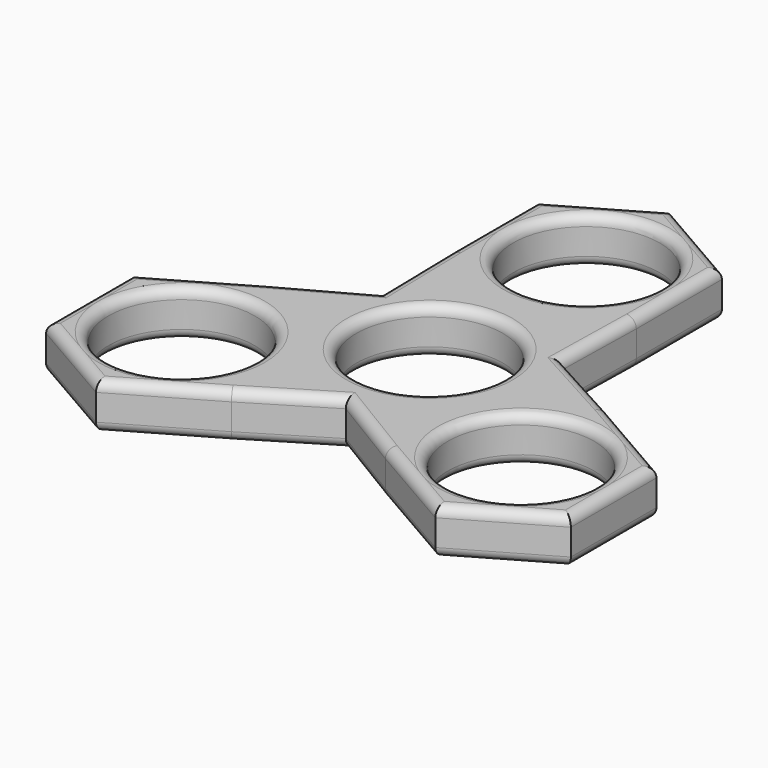
from build123d import *

# Parameters (mm, degrees)
F0_R         = 11.2
F1_DEPTH     = 7
F2_T1_DEPTH  = 23.8532758355
F2_T3_DEPTH  = 23.8532758355
F2_T5_DEPTH  = 23.8532758355
F2_T7_DEPTH  = 23.8532758355
F2_T9_DEPTH  = 23.8532758355
F2_T11_DEPTH = 23.8532758355
F2_T13_DEPTH = 23.8532758355
F2_T15_DEPTH = 23.8532758355
F2_T17_DEPTH = 23.8532758355
F2_T19_DEPTH = 23.8532758355
F2_T24_DEPTH = 21.2490117481
F2_T29_DEPTH = 21.2494848071
F2_T34_DEPTH = 21.2494848071
F2_T39_DEPTH = 21.2490117481
F2_T44_DEPTH = 21.249
F2_T49_DEPTH = 21.249
F2_T63_DEPTH = 21.2490117481
F2_T67_DEPTH = 21.2494848071
F2_T74_DEPTH = 21.2494848071
F2_T78_DEPTH = 21.2490117481
F2_T85_DEPTH = 21.249
F2_T89_DEPTH = 21.249
F3_T1_DEPTH  = 23.8532758355
F3_T3_DEPTH  = 23.8532758355
F3_T5_DEPTH  = 23.8532758355
F3_T7_DEPTH  = 23.8532758355
F3_T9_DEPTH  = 23.8532758355
F3_T11_DEPTH = 23.8532758355
F3_T13_DEPTH = 23.8532758355
F3_T15_DEPTH = 23.8532758355
F3_T17_DEPTH = 23.8532758355
F3_T19_DEPTH = 23.8532758355
F3_T24_DEPTH = 21.2490117481
F3_T29_DEPTH = 21.2494848071
F3_T34_DEPTH = 21.2494848071
F3_T39_DEPTH = 21.2490117481
F3_T44_DEPTH = 21.249
F3_T49_DEPTH = 21.249
F3_T63_DEPTH = 21.2494848071
F3_T67_DEPTH = 21.2490117481
F3_T74_DEPTH = 21.2490117481
F3_T78_DEPTH = 21.2494848071
F3_T85_DEPTH = 21.249
F3_T89_DEPTH = 21.249


# Not quite as in the source:
# - a fillet or chamfer that OpenCascade refuses, or shapes differently, is made with other operations: its cross-section is extruded or revolved along the edge and cut away or added


with BuildPart() as f1:
    # F0 (on Top) → F1 (new body)
    with BuildSketch(Plane.XY):
        Polygon((14.1623523086, 21.7544313529), (14.1623523086, 38.1077071884), (0, 46.2843451062), (-14.1623523086, 38.1077071884), (-14.1623523086, 21.7544313529), (-13.8703454286, 8.0080476669), (-25.9207897747, 1.388220244), (-40.0831420834, -6.7884176737), (-40.0831420834, -23.1416935092), (-25.9207897747, -31.318331427), (-11.7584374661, -23.1416935092), (0, -16.0160953339), (11.7584374661, -23.1416935092), (25.9207897747, -31.318331427), (40.0831420834, -23.1416935092), (40.0831420834, -6.7884176737), (25.9207897747, 1.388220244), (13.8703454286, 8.0080476669), align=None)
        with Locations((-25.9207897747, -14.9650555915)):
            Circle(F0_R, mode=Mode.SUBTRACT)
        Circle(F0_R, mode=Mode.SUBTRACT)
        with Locations((25.9207897747, -14.9650555915)):
            Circle(F0_R, mode=Mode.SUBTRACT)
        with Locations((0, 29.9310692707)):
            Circle(F0_R, mode=Mode.SUBTRACT)
    extrude(amount=F1_DEPTH)

    # F2: fillet of radius 1.5 on 22 edges, made by hand

    # F2_s2 → F2_t1 (cut)
    with BuildSketch(Plane(origin=(36.2494229052, -20.9286140723, 0), x_dir=(0, 0, 1), z_dir=(-0.8660254038, 0.5, 0))):
        with BuildLine():
            ThreePointArc((5.5, 14.1626288847), (6.5606601718, 13.7232890565), (7, 12.6626288847))
            Line((7, 12.6626288847), (7, 14.1626288847))
            Line((7, 14.1626288847), (5.5, 14.1626288847))
        make_face()
    extrude(amount=F2_T1_DEPTH, mode=Mode.SUBTRACT)

    # F2_s4 → F2_t3 (cut)
    with BuildSketch(Plane.XZ.offset(-41.8577071884)):
        with BuildLine():
            ThreePointArc((14.1623523086, 5.5), (13.7230124804, 6.5606601718), (12.6623523086, 7))
            Line((12.6623523086, 7), (14.1623523086, 7))
            Line((14.1623523086, 7), (14.1623523086, 5.5))
        make_face()
        with BuildLine():
            ThreePointArc((-14.1623523086, 5.5), (-13.7230124804, 6.5606601718), (-12.6623523086, 7))
            Line((-12.6623523086, 7), (-14.1623523086, 7))
            Line((-14.1623523086, 7), (-14.1623523086, 5.5))
        make_face()
    extrude(amount=F2_T3_DEPTH, mode=Mode.SUBTRACT)

    # F2_s6 → F2_t5 (cut)
    with BuildSketch(Plane(origin=(-2.6317617569, 1.5194483588, 0), x_dir=(0, 0, 1), z_dir=(-0.8660254038, 0.5, 0))):
        with BuildLine():
            ThreePointArc((5.5, 40.0834186595), (6.5606601718, 39.6440788312), (7, 38.5834186595))
            Line((7, 38.5834186595), (7, 40.0834186595))
            Line((7, 40.0834186595), (5.5, 40.0834186595))
        make_face()
    extrude(amount=F2_T5_DEPTH, mode=Mode.SUBTRACT)

    # F2_s8 → F2_t7 (cut)
    with BuildSketch(Plane(origin=(23.2893045939, 13.4460862765, 0), x_dir=(0, 0, 1), z_dir=(-0.8660254038, -0.5, 0))):
        with BuildLine():
            ThreePointArc((5.5, 40.0834186595), (6.5606601718, 39.6440788312), (7, 38.5834186595))
            Line((7, 38.5834186595), (7, 40.0834186595))
            Line((7, 40.0834186595), (5.5, 40.0834186595))
        make_face()
    extrude(amount=F2_T7_DEPTH, mode=Mode.SUBTRACT)

    # F2_s10 → F2_t9 (cut)
    with BuildSketch(Plane(origin=(-15.5918800682, -9.0019761545, 0), x_dir=(0, 0, 1), z_dir=(-0.8660254038, -0.5, 0))):
        with BuildLine():
            ThreePointArc((5.5, 14.1626288847), (6.5606601718, 13.7232890565), (7, 12.6626288847))
            Line((7, 12.6626288847), (7, 14.1626288847))
            Line((7, 14.1626288847), (5.5, 14.1626288847))
        make_face()
    extrude(amount=F2_T9_DEPTH, mode=Mode.SUBTRACT)

    # F2_s12 → F2_t11 (cut)
    with BuildSketch(Plane.XZ.offset(3.0384176737)):
        with BuildLine():
            ThreePointArc((-40.0831420834, 5.5), (-39.6438022551, 6.5606601718), (-38.5831420834, 7))
            Line((-38.5831420834, 7), (-40.0831420834, 7))
            Line((-40.0831420834, 7), (-40.0831420834, 5.5))
        make_face()
        with BuildLine():
            ThreePointArc((40.0831420834, 5.5), (39.6438022551, 6.5606601718), (38.5831420834, 7))
            Line((38.5831420834, 7), (40.0831420834, 7))
            Line((40.0831420834, 7), (40.0831420834, 5.5))
        make_face()
    extrude(amount=F2_T11_DEPTH, mode=Mode.SUBTRACT)

    # F2_s14 → F2_t13 (cut)
    with BuildSketch(Plane(origin=(-23.2893045939, 13.4460862765, 0), x_dir=(0, 0, 1), z_dir=(0.8660254038, -0.5, 0))):
        with BuildLine():
            ThreePointArc((5.5, 40.0828655072), (6.5606601718, 39.643525679), (7, 38.5828655072))
            Line((7, 38.5828655072), (7, 40.0828655072))
            Line((7, 40.0828655072), (5.5, 40.0828655072))
        make_face()
    extrude(amount=F2_T13_DEPTH, mode=Mode.SUBTRACT)

    # F2_s16 → F2_t15 (cut)
    with BuildSketch(Plane(origin=(-36.2494229052, -20.9286140723, 0), x_dir=(0, 0, 1), z_dir=(0.8660254038, 0.5, 0))):
        with BuildLine():
            ThreePointArc((5.5, 14.1620757325), (6.5606601718, 13.7227359043), (7, 12.6620757325))
            Line((7, 12.6620757325), (7, 14.1620757325))
            Line((7, 14.1620757325), (5.5, 14.1620757325))
        make_face()
    extrude(amount=F2_T15_DEPTH, mode=Mode.SUBTRACT)

    # F2_s18 → F2_t17 (cut)
    with BuildSketch(Plane(origin=(15.5918800682, -9.0019761545, 0), x_dir=(0, 0, 1), z_dir=(0.8660254038, -0.5, 0))):
        with BuildLine():
            ThreePointArc((5.5, 14.1620757325), (6.5606601718, 13.7227359043), (7, 12.6620757325))
            Line((7, 12.6620757325), (7, 14.1620757325))
            Line((7, 14.1620757325), (5.5, 14.1620757325))
        make_face()
    extrude(amount=F2_T17_DEPTH, mode=Mode.SUBTRACT)

    # F2_s20 → F2_t19 (cut)
    with BuildSketch(Plane(origin=(2.6317617569, 1.5194483588, 0), x_dir=(0, 0, 1), z_dir=(0.8660254038, 0.5, 0))):
        with BuildLine():
            ThreePointArc((5.5, 40.0828655072), (6.5606601718, 39.643525679), (7, 38.5828655072))
            Line((7, 38.5828655072), (7, 40.0828655072))
            Line((7, 40.0828655072), (5.5, 40.0828655072))
        make_face()
    extrude(amount=F2_T19_DEPTH, mode=Mode.SUBTRACT)


with BuildPart() as f2_tool22:
    # F2_s23 → F2_t24 (new body)
    with BuildSketch(Plane(origin=(22.6127394317, -12.422150445, 0), x_dir=(0, 0, 1), z_dir=(-0.8764589461, 0.4814765995, 0))):
        with BuildLine():
            ThreePointArc((5.5, 13.696971769), (6.5606601718, 13.2576319408), (7, 12.196971769))
            Line((7, 12.196971769), (7, 13.696971769))
            Line((7, 13.696971769), (5.5, 13.696971769))
        make_face()
    extrude(amount=F2_T24_DEPTH)

    split(bisect_by=Plane(origin=(13.6940555403, -0.290895302, 0), x_dir=(0, 0, 1), z_dir=(0.9997744555, -0.0212376597, 0)), keep=Keep.TOP)


with BuildPart() as f1_1:
    add(f1.part)

    # F2_t21: cut F2_tool22
    add(f2_tool22.part, mode=Mode.SUBTRACT)


with BuildPart() as f2_tool27:
    # F2_s28 → F2_t29 (new body)
    with BuildSketch(Plane(origin=(0.0966486642, 4.5497887609, 0), x_dir=(0, 0, 1), z_dir=(0.0212376597, 0.9997744555, 0))):
        with BuildLine():
            ThreePointArc((5.5, 13.6971448564), (6.5606601718, 13.2578050282), (7, 12.1971448564))
            Line((7, 12.1971448564), (7, 13.6971448564))
            Line((7, 13.6971448564), (5.5, 13.6971448564))
        make_face()
    extrude(amount=F2_T29_DEPTH)

    split(bisect_by=Plane(origin=(6.5947713908, 12.0048334409, 0), x_dir=(0, 0, 1), z_dir=(0.4814765995, 0.8764589461, 0)), keep=Keep.TOP)


with BuildPart() as f1_2:
    add(f1_1.part)

    # F2_t26: cut F2_tool27
    add(f2_tool27.part, mode=Mode.SUBTRACT)


with BuildPart() as f2_tool32:
    # F2_s33 → F2_t34 (new body)
    with BuildSketch(Plane(origin=(-0.5479379924, 25.7944808629, 0), x_dir=(0, 0, 1), z_dir=(0.0212376597, -0.9997744555, 0))):
        with BuildLine():
            ThreePointArc((5.5, 13.6971448564), (6.5606601718, 13.2578050282), (7, 12.1971448564))
            Line((7, 12.1971448564), (7, 13.6971448564))
            Line((7, 13.6971448564), (5.5, 13.6971448564))
        make_face()
    extrude(amount=F2_T34_DEPTH)

    split(bisect_by=Plane(origin=(-6.5947713908, 12.0048334409, 0), x_dir=(0, 0, 1), z_dir=(-0.4814765995, 0.8764589461, 0)), keep=Keep.TOP)


with BuildPart() as f1_3:
    add(f1_2.part)

    # F2_t31: cut F2_tool32
    add(f2_tool32.part, mode=Mode.SUBTRACT)


with BuildPart() as f2_tool37:
    # F2_s38 → F2_t39 (new body)
    with BuildSketch(Plane(origin=(-3.9888529901, -2.1912485259, 0), x_dir=(0, 0, 1), z_dir=(-0.8764589461, -0.4814765995, 0))):
        with BuildLine():
            ThreePointArc((5.5, 13.696971769), (6.5606601718, 13.2576319408), (7, 12.196971769))
            Line((7, 12.196971769), (7, 13.696971769))
            Line((7, 13.696971769), (5.5, 13.696971769))
        make_face()
    extrude(amount=F2_T39_DEPTH)

    split(bisect_by=Plane(origin=(-13.6940555403, -0.290895302, 0), x_dir=(0, 0, 1), z_dir=(-0.9997744555, -0.0212376597, 0)), keep=Keep.TOP)


with BuildPart() as f1_4:
    add(f1_3.part)

    # F2_t36: cut F2_tool37
    add(f2_tool37.part, mode=Mode.SUBTRACT)


with BuildPart() as f2_tool42:
    # F2_s43 → F2_t44 (new body)
    with BuildSketch(Plane(origin=(-22.0643241976, -13.3709524497, 0), x_dir=(0, 0, 1), z_dir=(0.8552212864, 0.5182630137, 0))):
        with BuildLine():
            ThreePointArc((5.5, 13.6973056538), (6.5606601718, 13.2579658256), (7, 12.1973056538))
            Line((7, 12.1973056538), (7, 13.6973056538))
            Line((7, 13.6973056538), (5.5, 13.6973056538))
        make_face()
    extrude(amount=F2_T44_DEPTH)

    split(bisect_by=Plane(origin=(-7.0988069077, -11.7142273609, 0), x_dir=(0, 0, 1), z_dir=(-0.5182630137, -0.8552212864, 0)), keep=Keep.TOP)


with BuildPart() as f1_5:
    add(f1_4.part)

    # F2_t41: cut F2_tool42
    add(f2_tool42.part, mode=Mode.SUBTRACT)


with BuildPart() as f2_tool47:
    # F2_s48 → F2_t49 (new body)
    with BuildSketch(Plane(origin=(3.8917270838, -2.3583816717, 0), x_dir=(0, 0, 1), z_dir=(0.8552212864, -0.5182630137, 0))):
        with BuildLine():
            ThreePointArc((5.5, 13.6973056538), (6.5606601718, 13.2579658256), (7, 12.1973056538))
            Line((7, 12.1973056538), (7, 13.6973056538))
            Line((7, 13.6973056538), (5.5, 13.6973056538))
        make_face()
    extrude(amount=F2_T49_DEPTH)

    split(bisect_by=Plane(origin=(7.0988069077, -11.7142273609, 0), x_dir=(0, 0, 1), z_dir=(0.5182630137, -0.8552212864, 0)), keep=Keep.TOP)


with BuildPart() as f1_6:
    add(f1_5.part)

    # F2_t46: cut F2_tool47
    add(f2_tool47.part, mode=Mode.SUBTRACT)

    # F2_s51 → F2_t52 (revolve, cut)
    with BuildSketch(Plane.XZ.offset(14.9650555915)):
        with BuildLine():
            ThreePointArc((-14.7207897747, 5.5), (-14.2814499465, 6.5606601718), (-13.2207897747, 7))
            Line((-13.2207897747, 7), (-14.7207897747, 7))
            Line((-14.7207897747, 7), (-14.7207897747, 5.5))
        make_face()
    revolve(axis=Axis((-25.9207897747, -14.9650555915, 7), (0, 0, 1)), mode=Mode.SUBTRACT)

    # F2_s53 → F2_t54 (revolve, cut)
    with BuildSketch(Plane.XZ):
        with BuildLine():
            ThreePointArc((11.2, 5.5), (11.6393398282, 6.5606601718), (12.7, 7))
            Line((12.7, 7), (11.2, 7))
            Line((11.2, 7), (11.2, 5.5))
        make_face()
    revolve(axis=Axis((0, 0, 7), (0, 0, 1)), mode=Mode.SUBTRACT)

    # F2_s55 → F2_t56 (revolve, cut)
    with BuildSketch(Plane.XZ.offset(14.9650555915)):
        with BuildLine():
            ThreePointArc((37.1207897747, 5.5), (37.5601296029, 6.5606601718), (38.6207897747, 7))
            Line((38.6207897747, 7), (37.1207897747, 7))
            Line((37.1207897747, 7), (37.1207897747, 5.5))
        make_face()
    revolve(axis=Axis((25.9207897747, -14.9650555915, 7), (0, 0, 1)), mode=Mode.SUBTRACT)

    # F2_s57 → F2_t58 (revolve, cut)
    with BuildSketch(Plane.XZ.offset(-29.9310692707)):
        with BuildLine():
            ThreePointArc((11.2, 5.5), (11.6393398282, 6.5606601718), (12.7, 7))
            Line((12.7, 7), (11.2, 7))
            Line((11.2, 7), (11.2, 5.5))
        make_face()
    revolve(axis=Axis((0, 29.9310692707, 7), (0, 0, 1)), mode=Mode.SUBTRACT)


with BuildPart() as f2_tool61:
    # F2_s62 → F2_t63 (new body)
    with BuildSketch(Plane(origin=(22.6127394317, -12.422150445, 0), x_dir=(0, 0, 1), z_dir=(-0.8764589461, 0.4814765995, 0))):
        with BuildLine():
            ThreePointArc((5.5, 13.696971769), (6.5606601718, 13.2576319408), (7, 12.196971769))
            Line((7, 12.196971769), (7, 13.696971769))
            Line((7, 13.696971769), (5.5, 13.696971769))
        make_face()
    extrude(amount=F2_T63_DEPTH)

    split(bisect_by=Plane(origin=(13.6940555403, -0.290895302, 0), x_dir=(0, 0, 1), z_dir=(-0.9997744555, 0.0212376597, 0)), keep=Keep.TOP)


with BuildPart() as f2_tool65:
    # F2_s66 → F2_t67 (new body)
    with BuildSketch(Plane(origin=(0.0966486642, 4.5497887609, 0), x_dir=(0, 0, 1), z_dir=(0.0212376597, 0.9997744555, 0))):
        with BuildLine():
            ThreePointArc((5.5, 13.6971448564), (6.5606601718, 13.2578050282), (7, 12.1971448564))
            Line((7, 12.1971448564), (7, 13.6971448564))
            Line((7, 13.6971448564), (5.5, 13.6971448564))
        make_face()
    extrude(amount=F2_T67_DEPTH)

    split(bisect_by=Plane(origin=(6.5947713908, 12.0048334409, 0), x_dir=(0, 0, 1), z_dir=(-0.4814765995, -0.8764589461, 0)), keep=Keep.TOP)


with BuildPart() as f2_tool61_1:
    add(f2_tool61.part)

    # F2_t69: intersect F2_tool65
    add(f2_tool65.part, mode=Mode.INTERSECT)


with BuildPart() as f1_7:
    add(f1_6.part)

    # F2_t59: cut F2_tool61
    add(f2_tool61_1.part, mode=Mode.SUBTRACT)


with BuildPart() as f2_tool72:
    # F2_s73 → F2_t74 (new body)
    with BuildSketch(Plane(origin=(-0.5479379924, 25.7944808629, 0), x_dir=(0, 0, 1), z_dir=(0.0212376597, -0.9997744555, 0))):
        with BuildLine():
            ThreePointArc((5.5, 13.6971448564), (6.5606601718, 13.2578050282), (7, 12.1971448564))
            Line((7, 12.1971448564), (7, 13.6971448564))
            Line((7, 13.6971448564), (5.5, 13.6971448564))
        make_face()
    extrude(amount=F2_T74_DEPTH)

    split(bisect_by=Plane(origin=(-6.5947713908, 12.0048334409, 0), x_dir=(0, 0, 1), z_dir=(0.4814765995, -0.8764589461, 0)), keep=Keep.TOP)


with BuildPart() as f2_tool76:
    # F2_s77 → F2_t78 (new body)
    with BuildSketch(Plane(origin=(-3.9888529901, -2.1912485259, 0), x_dir=(0, 0, 1), z_dir=(-0.8764589461, -0.4814765995, 0))):
        with BuildLine():
            ThreePointArc((5.5, 13.696971769), (6.5606601718, 13.2576319408), (7, 12.196971769))
            Line((7, 12.196971769), (7, 13.696971769))
            Line((7, 13.696971769), (5.5, 13.696971769))
        make_face()
    extrude(amount=F2_T78_DEPTH)

    split(bisect_by=Plane(origin=(-13.6940555403, -0.290895302, 0), x_dir=(0, 0, 1), z_dir=(0.9997744555, 0.0212376597, 0)), keep=Keep.TOP)


with BuildPart() as f2_tool72_1:
    add(f2_tool72.part)

    # F2_t80: intersect F2_tool76
    add(f2_tool76.part, mode=Mode.INTERSECT)


with BuildPart() as f1_8:
    add(f1_7.part)

    # F2_t70: cut F2_tool72
    add(f2_tool72_1.part, mode=Mode.SUBTRACT)


with BuildPart() as f2_tool83:
    # F2_s84 → F2_t85 (new body)
    with BuildSketch(Plane(origin=(-22.0643241976, -13.3709524497, 0), x_dir=(0, 0, 1), z_dir=(0.8552212864, 0.5182630137, 0))):
        with BuildLine():
            ThreePointArc((5.5, 13.6973056538), (6.5606601718, 13.2579658256), (7, 12.1973056538))
            Line((7, 12.1973056538), (7, 13.6973056538))
            Line((7, 13.6973056538), (5.5, 13.6973056538))
        make_face()
    extrude(amount=F2_T85_DEPTH)

    split(bisect_by=Plane(origin=(-7.0988069077, -11.7142273609, 0), x_dir=(0, 0, 1), z_dir=(0.5182630137, 0.8552212864, 0)), keep=Keep.TOP)


with BuildPart() as f2_tool87:
    # F2_s88 → F2_t89 (new body)
    with BuildSketch(Plane(origin=(3.8917270838, -2.3583816717, 0), x_dir=(0, 0, 1), z_dir=(0.8552212864, -0.5182630137, 0))):
        with BuildLine():
            ThreePointArc((5.5, 13.6973056538), (6.5606601718, 13.2579658256), (7, 12.1973056538))
            Line((7, 12.1973056538), (7, 13.6973056538))
            Line((7, 13.6973056538), (5.5, 13.6973056538))
        make_face()
    extrude(amount=F2_T89_DEPTH)

    split(bisect_by=Plane(origin=(7.0988069077, -11.7142273609, 0), x_dir=(0, 0, 1), z_dir=(-0.5182630137, 0.8552212864, 0)), keep=Keep.TOP)


with BuildPart() as f2_tool83_1:
    add(f2_tool83.part)

    # F2_t91: intersect F2_tool87
    add(f2_tool87.part, mode=Mode.INTERSECT)


with BuildPart() as f1_9:
    add(f1_8.part)

    # F2_t81: cut F2_tool83
    add(f2_tool83_1.part, mode=Mode.SUBTRACT)

    # F3: fillet of radius 1.5 on 22 edges, made by hand

    # F3_s2 → F3_t1 (cut)
    with BuildSketch(Plane(origin=(36.2494229052, -20.9286140723, 0), x_dir=(0, 0, 1), z_dir=(-0.8660254038, 0.5, 0))):
        with BuildLine():
            ThreePointArc((1.5, 14.1626288847), (0.4393398282, 13.7232890565), (0, 12.6626288847))
            Line((0, 12.6626288847), (0, 14.1626288847))
            Line((0, 14.1626288847), (1.5, 14.1626288847))
        make_face()
    extrude(amount=F3_T1_DEPTH, mode=Mode.SUBTRACT)

    # F3_s4 → F3_t3 (cut)
    with BuildSketch(Plane.XZ.offset(-41.8577071884)):
        with BuildLine():
            ThreePointArc((14.1623523086, 1.5), (13.7230124804, 0.4393398282), (12.6623523086, 0))
            Line((12.6623523086, 0), (14.1623523086, 0))
            Line((14.1623523086, 0), (14.1623523086, 1.5))
        make_face()
        with BuildLine():
            ThreePointArc((-14.1623523086, 1.5), (-13.7230124804, 0.4393398282), (-12.6623523086, 0))
            Line((-12.6623523086, 0), (-14.1623523086, 0))
            Line((-14.1623523086, 0), (-14.1623523086, 1.5))
        make_face()
    extrude(amount=F3_T3_DEPTH, mode=Mode.SUBTRACT)

    # F3_s6 → F3_t5 (cut)
    with BuildSketch(Plane(origin=(-2.6317617569, 1.5194483588, 0), x_dir=(0, 0, 1), z_dir=(-0.8660254038, 0.5, 0))):
        with BuildLine():
            ThreePointArc((1.5, 40.0834186595), (0.4393398282, 39.6440788312), (0, 38.5834186595))
            Line((0, 38.5834186595), (0, 40.0834186595))
            Line((0, 40.0834186595), (1.5, 40.0834186595))
        make_face()
    extrude(amount=F3_T5_DEPTH, mode=Mode.SUBTRACT)

    # F3_s8 → F3_t7 (cut)
    with BuildSketch(Plane(origin=(23.2893045939, 13.4460862765, 0), x_dir=(0, 0, 1), z_dir=(-0.8660254038, -0.5, 0))):
        with BuildLine():
            ThreePointArc((1.5, 40.0834186595), (0.4393398282, 39.6440788312), (0, 38.5834186595))
            Line((0, 38.5834186595), (0, 40.0834186595))
            Line((0, 40.0834186595), (1.5, 40.0834186595))
        make_face()
    extrude(amount=F3_T7_DEPTH, mode=Mode.SUBTRACT)

    # F3_s10 → F3_t9 (cut)
    with BuildSketch(Plane(origin=(-15.5918800682, -9.0019761545, 0), x_dir=(0, 0, 1), z_dir=(-0.8660254038, -0.5, 0))):
        with BuildLine():
            ThreePointArc((1.5, 14.1626288847), (0.4393398282, 13.7232890565), (0, 12.6626288847))
            Line((0, 12.6626288847), (0, 14.1626288847))
            Line((0, 14.1626288847), (1.5, 14.1626288847))
        make_face()
    extrude(amount=F3_T9_DEPTH, mode=Mode.SUBTRACT)

    # F3_s12 → F3_t11 (cut)
    with BuildSketch(Plane.XZ.offset(3.0384176737)):
        with BuildLine():
            ThreePointArc((-40.0831420834, 1.5), (-39.6438022551, 0.4393398282), (-38.5831420834, 0))
            Line((-38.5831420834, 0), (-40.0831420834, 0))
            Line((-40.0831420834, 0), (-40.0831420834, 1.5))
        make_face()
        with BuildLine():
            ThreePointArc((40.0831420834, 1.5), (39.6438022551, 0.4393398282), (38.5831420834, 0))
            Line((38.5831420834, 0), (40.0831420834, 0))
            Line((40.0831420834, 0), (40.0831420834, 1.5))
        make_face()
    extrude(amount=F3_T11_DEPTH, mode=Mode.SUBTRACT)

    # F3_s14 → F3_t13 (cut)
    with BuildSketch(Plane(origin=(-23.2893045939, 13.4460862765, 0), x_dir=(0, 0, 1), z_dir=(0.8660254038, -0.5, 0))):
        with BuildLine():
            ThreePointArc((1.5, 40.0828655072), (0.4393398282, 39.643525679), (0, 38.5828655072))
            Line((0, 38.5828655072), (0, 40.0828655072))
            Line((0, 40.0828655072), (1.5, 40.0828655072))
        make_face()
    extrude(amount=F3_T13_DEPTH, mode=Mode.SUBTRACT)

    # F3_s16 → F3_t15 (cut)
    with BuildSketch(Plane(origin=(-36.2494229052, -20.9286140723, 0), x_dir=(0, 0, 1), z_dir=(0.8660254038, 0.5, 0))):
        with BuildLine():
            ThreePointArc((1.5, 14.1620757325), (0.4393398282, 13.7227359043), (0, 12.6620757325))
            Line((0, 12.6620757325), (0, 14.1620757325))
            Line((0, 14.1620757325), (1.5, 14.1620757325))
        make_face()
    extrude(amount=F3_T15_DEPTH, mode=Mode.SUBTRACT)

    # F3_s18 → F3_t17 (cut)
    with BuildSketch(Plane(origin=(15.5918800682, -9.0019761545, 0), x_dir=(0, 0, 1), z_dir=(0.8660254038, -0.5, 0))):
        with BuildLine():
            ThreePointArc((1.5, 14.1620757325), (0.4393398282, 13.7227359043), (0, 12.6620757325))
            Line((0, 12.6620757325), (0, 14.1620757325))
            Line((0, 14.1620757325), (1.5, 14.1620757325))
        make_face()
    extrude(amount=F3_T17_DEPTH, mode=Mode.SUBTRACT)

    # F3_s20 → F3_t19 (cut)
    with BuildSketch(Plane(origin=(2.6317617569, 1.5194483588, 0), x_dir=(0, 0, 1), z_dir=(0.8660254038, 0.5, 0))):
        with BuildLine():
            ThreePointArc((1.5, 40.0828655072), (0.4393398282, 39.643525679), (0, 38.5828655072))
            Line((0, 38.5828655072), (0, 40.0828655072))
            Line((0, 40.0828655072), (1.5, 40.0828655072))
        make_face()
    extrude(amount=F3_T19_DEPTH, mode=Mode.SUBTRACT)


with BuildPart() as f3_tool22:
    # F3_s23 → F3_t24 (new body)
    with BuildSketch(Plane(origin=(22.6127394317, -12.422150445, 0), x_dir=(0, 0, 1), z_dir=(-0.8764589461, 0.4814765995, 0))):
        with BuildLine():
            ThreePointArc((1.5, 13.696971769), (0.4393398282, 13.2576319408), (0, 12.196971769))
            Line((0, 12.196971769), (0, 13.696971769))
            Line((0, 13.696971769), (1.5, 13.696971769))
        make_face()
    extrude(amount=F3_T24_DEPTH)

    split(bisect_by=Plane(origin=(13.6940555403, -0.290895302, 0), x_dir=(0, 0, 1), z_dir=(0.9997744555, -0.0212376597, 0)), keep=Keep.TOP)


with BuildPart() as f1_10:
    add(f1_9.part)

    # F3_t21: cut F3_tool22
    add(f3_tool22.part, mode=Mode.SUBTRACT)


with BuildPart() as f3_tool27:
    # F3_s28 → F3_t29 (new body)
    with BuildSketch(Plane(origin=(0.0966486642, 4.5497887609, 0), x_dir=(0, 0, 1), z_dir=(0.0212376597, 0.9997744555, 0))):
        with BuildLine():
            ThreePointArc((1.5, 13.6971448564), (0.4393398282, 13.2578050282), (0, 12.1971448564))
            Line((0, 12.1971448564), (0, 13.6971448564))
            Line((0, 13.6971448564), (1.5, 13.6971448564))
        make_face()
    extrude(amount=F3_T29_DEPTH)

    split(bisect_by=Plane(origin=(6.5947713908, 12.0048334409, 0), x_dir=(0, 0, 1), z_dir=(0.4814765995, 0.8764589461, 0)), keep=Keep.TOP)


with BuildPart() as f1_11:
    add(f1_10.part)

    # F3_t26: cut F3_tool27
    add(f3_tool27.part, mode=Mode.SUBTRACT)


with BuildPart() as f3_tool32:
    # F3_s33 → F3_t34 (new body)
    with BuildSketch(Plane(origin=(-0.5479379924, 25.7944808629, 0), x_dir=(0, 0, 1), z_dir=(0.0212376597, -0.9997744555, 0))):
        with BuildLine():
            ThreePointArc((1.5, 13.6971448564), (0.4393398282, 13.2578050282), (0, 12.1971448564))
            Line((0, 12.1971448564), (0, 13.6971448564))
            Line((0, 13.6971448564), (1.5, 13.6971448564))
        make_face()
    extrude(amount=F3_T34_DEPTH)

    split(bisect_by=Plane(origin=(-6.5947713908, 12.0048334409, 0), x_dir=(0, 0, 1), z_dir=(-0.4814765995, 0.8764589461, 0)), keep=Keep.TOP)


with BuildPart() as f1_12:
    add(f1_11.part)

    # F3_t31: cut F3_tool32
    add(f3_tool32.part, mode=Mode.SUBTRACT)


with BuildPart() as f3_tool37:
    # F3_s38 → F3_t39 (new body)
    with BuildSketch(Plane(origin=(-3.9888529901, -2.1912485259, 0), x_dir=(0, 0, 1), z_dir=(-0.8764589461, -0.4814765995, 0))):
        with BuildLine():
            ThreePointArc((1.5, 13.696971769), (0.4393398282, 13.2576319408), (0, 12.196971769))
            Line((0, 12.196971769), (0, 13.696971769))
            Line((0, 13.696971769), (1.5, 13.696971769))
        make_face()
    extrude(amount=F3_T39_DEPTH)

    split(bisect_by=Plane(origin=(-13.6940555403, -0.290895302, 0), x_dir=(0, 0, 1), z_dir=(-0.9997744555, -0.0212376597, 0)), keep=Keep.TOP)


with BuildPart() as f1_13:
    add(f1_12.part)

    # F3_t36: cut F3_tool37
    add(f3_tool37.part, mode=Mode.SUBTRACT)


with BuildPart() as f3_tool42:
    # F3_s43 → F3_t44 (new body)
    with BuildSketch(Plane(origin=(-22.0643241976, -13.3709524497, 0), x_dir=(0, 0, 1), z_dir=(0.8552212864, 0.5182630137, 0))):
        with BuildLine():
            ThreePointArc((1.5, 13.6973056538), (0.4393398282, 13.2579658256), (0, 12.1973056538))
            Line((0, 12.1973056538), (0, 13.6973056538))
            Line((0, 13.6973056538), (1.5, 13.6973056538))
        make_face()
    extrude(amount=F3_T44_DEPTH)

    split(bisect_by=Plane(origin=(-7.0988069077, -11.7142273609, 0), x_dir=(0, 0, 1), z_dir=(-0.5182630137, -0.8552212864, 0)), keep=Keep.TOP)


with BuildPart() as f1_14:
    add(f1_13.part)

    # F3_t41: cut F3_tool42
    add(f3_tool42.part, mode=Mode.SUBTRACT)


with BuildPart() as f3_tool47:
    # F3_s48 → F3_t49 (new body)
    with BuildSketch(Plane(origin=(3.8917270838, -2.3583816717, 0), x_dir=(0, 0, 1), z_dir=(0.8552212864, -0.5182630137, 0))):
        with BuildLine():
            ThreePointArc((1.5, 13.6973056538), (0.4393398282, 13.2579658256), (0, 12.1973056538))
            Line((0, 12.1973056538), (0, 13.6973056538))
            Line((0, 13.6973056538), (1.5, 13.6973056538))
        make_face()
    extrude(amount=F3_T49_DEPTH)

    split(bisect_by=Plane(origin=(7.0988069077, -11.7142273609, 0), x_dir=(0, 0, 1), z_dir=(0.5182630137, -0.8552212864, 0)), keep=Keep.TOP)


with BuildPart() as f1_15:
    add(f1_14.part)

    # F3_t46: cut F3_tool47
    add(f3_tool47.part, mode=Mode.SUBTRACT)

    # F3_s51 → F3_t52 (revolve, cut)
    with BuildSketch(Plane.XZ.offset(14.9650555915)):
        with BuildLine():
            ThreePointArc((-14.7207897747, 1.5), (-14.2814499465, 0.4393398282), (-13.2207897747, 0))
            Line((-13.2207897747, 0), (-14.7207897747, 0))
            Line((-14.7207897747, 0), (-14.7207897747, 1.5))
        make_face()
    revolve(axis=Axis((-25.9207897747, -14.9650555915, 0), (0, 0, 1)), mode=Mode.SUBTRACT)

    # F3_s53 → F3_t54 (revolve, cut)
    with BuildSketch(Plane.XZ):
        with BuildLine():
            ThreePointArc((11.2, 1.5), (11.6393398282, 0.4393398282), (12.7, 0))
            Line((12.7, 0), (11.2, 0))
            Line((11.2, 0), (11.2, 1.5))
        make_face()
    revolve(axis=Axis((0, 0, 0), (0, 0, 1)), mode=Mode.SUBTRACT)

    # F3_s55 → F3_t56 (revolve, cut)
    with BuildSketch(Plane.XZ.offset(14.9650555915)):
        with BuildLine():
            ThreePointArc((37.1207897747, 1.5), (37.5601296029, 0.4393398282), (38.6207897747, 0))
            Line((38.6207897747, 0), (37.1207897747, 0))
            Line((37.1207897747, 0), (37.1207897747, 1.5))
        make_face()
    revolve(axis=Axis((25.9207897747, -14.9650555915, 0), (0, 0, 1)), mode=Mode.SUBTRACT)

    # F3_s57 → F3_t58 (revolve, cut)
    with BuildSketch(Plane.XZ.offset(-29.9310692707)):
        with BuildLine():
            ThreePointArc((11.2, 1.5), (11.6393398282, 0.4393398282), (12.7, 0))
            Line((12.7, 0), (11.2, 0))
            Line((11.2, 0), (11.2, 1.5))
        make_face()
    revolve(axis=Axis((0, 29.9310692707, 0), (0, 0, 1)), mode=Mode.SUBTRACT)


with BuildPart() as f3_tool61:
    # F3_s62 → F3_t63 (new body)
    with BuildSketch(Plane(origin=(0.0966486642, 4.5497887609, 0), x_dir=(0, 0, 1), z_dir=(0.0212376597, 0.9997744555, 0))):
        with BuildLine():
            ThreePointArc((1.5, 13.6971448564), (0.4393398282, 13.2578050282), (0, 12.1971448564))
            Line((0, 12.1971448564), (0, 13.6971448564))
            Line((0, 13.6971448564), (1.5, 13.6971448564))
        make_face()
    extrude(amount=F3_T63_DEPTH)

    split(bisect_by=Plane(origin=(6.5947713908, 12.0048334409, 0), x_dir=(0, 0, 1), z_dir=(-0.4814765995, -0.8764589461, 0)), keep=Keep.TOP)


with BuildPart() as f3_tool65:
    # F3_s66 → F3_t67 (new body)
    with BuildSketch(Plane(origin=(22.6127394317, -12.422150445, 0), x_dir=(0, 0, 1), z_dir=(-0.8764589461, 0.4814765995, 0))):
        with BuildLine():
            ThreePointArc((1.5, 13.696971769), (0.4393398282, 13.2576319408), (0, 12.196971769))
            Line((0, 12.196971769), (0, 13.696971769))
            Line((0, 13.696971769), (1.5, 13.696971769))
        make_face()
    extrude(amount=F3_T67_DEPTH)

    split(bisect_by=Plane(origin=(13.6940555403, -0.290895302, 0), x_dir=(0, 0, 1), z_dir=(-0.9997744555, 0.0212376597, 0)), keep=Keep.TOP)


with BuildPart() as f3_tool61_1:
    add(f3_tool61.part)

    # F3_t69: intersect F3_tool65
    add(f3_tool65.part, mode=Mode.INTERSECT)


with BuildPart() as f1_16:
    add(f1_15.part)

    # F3_t59: cut F3_tool61
    add(f3_tool61_1.part, mode=Mode.SUBTRACT)


with BuildPart() as f3_tool72:
    # F3_s73 → F3_t74 (new body)
    with BuildSketch(Plane(origin=(-3.9888529901, -2.1912485259, 0), x_dir=(0, 0, 1), z_dir=(-0.8764589461, -0.4814765995, 0))):
        with BuildLine():
            ThreePointArc((1.5, 13.696971769), (0.4393398282, 13.2576319408), (0, 12.196971769))
            Line((0, 12.196971769), (0, 13.696971769))
            Line((0, 13.696971769), (1.5, 13.696971769))
        make_face()
    extrude(amount=F3_T74_DEPTH)

    split(bisect_by=Plane(origin=(-13.6940555403, -0.290895302, 0), x_dir=(0, 0, 1), z_dir=(0.9997744555, 0.0212376597, 0)), keep=Keep.TOP)


with BuildPart() as f3_tool76:
    # F3_s77 → F3_t78 (new body)
    with BuildSketch(Plane(origin=(-0.5479379924, 25.7944808629, 0), x_dir=(0, 0, 1), z_dir=(0.0212376597, -0.9997744555, 0))):
        with BuildLine():
            ThreePointArc((1.5, 13.6971448564), (0.4393398282, 13.2578050282), (0, 12.1971448564))
            Line((0, 12.1971448564), (0, 13.6971448564))
            Line((0, 13.6971448564), (1.5, 13.6971448564))
        make_face()
    extrude(amount=F3_T78_DEPTH)

    split(bisect_by=Plane(origin=(-6.5947713908, 12.0048334409, 0), x_dir=(0, 0, 1), z_dir=(0.4814765995, -0.8764589461, 0)), keep=Keep.TOP)


with BuildPart() as f3_tool72_1:
    add(f3_tool72.part)

    # F3_t80: intersect F3_tool76
    add(f3_tool76.part, mode=Mode.INTERSECT)


with BuildPart() as f1_17:
    add(f1_16.part)

    # F3_t70: cut F3_tool72
    add(f3_tool72_1.part, mode=Mode.SUBTRACT)


with BuildPart() as f3_tool83:
    # F3_s84 → F3_t85 (new body)
    with BuildSketch(Plane(origin=(3.8917270838, -2.3583816717, 0), x_dir=(0, 0, 1), z_dir=(0.8552212864, -0.5182630137, 0))):
        with BuildLine():
            ThreePointArc((1.5, 13.6973056538), (0.4393398282, 13.2579658256), (0, 12.1973056538))
            Line((0, 12.1973056538), (0, 13.6973056538))
            Line((0, 13.6973056538), (1.5, 13.6973056538))
        make_face()
    extrude(amount=F3_T85_DEPTH)

    split(bisect_by=Plane(origin=(7.0988069077, -11.7142273609, 0), x_dir=(0, 0, 1), z_dir=(-0.5182630137, 0.8552212864, 0)), keep=Keep.TOP)


with BuildPart() as f3_tool87:
    # F3_s88 → F3_t89 (new body)
    with BuildSketch(Plane(origin=(-22.0643241976, -13.3709524497, 0), x_dir=(0, 0, 1), z_dir=(0.8552212864, 0.5182630137, 0))):
        with BuildLine():
            ThreePointArc((1.5, 13.6973056538), (0.4393398282, 13.2579658256), (0, 12.1973056538))
            Line((0, 12.1973056538), (0, 13.6973056538))
            Line((0, 13.6973056538), (1.5, 13.6973056538))
        make_face()
    extrude(amount=F3_T89_DEPTH)

    split(bisect_by=Plane(origin=(-7.0988069077, -11.7142273609, 0), x_dir=(0, 0, 1), z_dir=(0.5182630137, 0.8552212864, 0)), keep=Keep.TOP)


with BuildPart() as f3_tool83_1:
    add(f3_tool83.part)

    # F3_t91: intersect F3_tool87
    add(f3_tool87.part, mode=Mode.INTERSECT)


with BuildPart() as f1_18:
    add(f1_17.part)

    # F3_t81: cut F3_tool83
    add(f3_tool83_1.part, mode=Mode.SUBTRACT)


solid = f1_18.part
